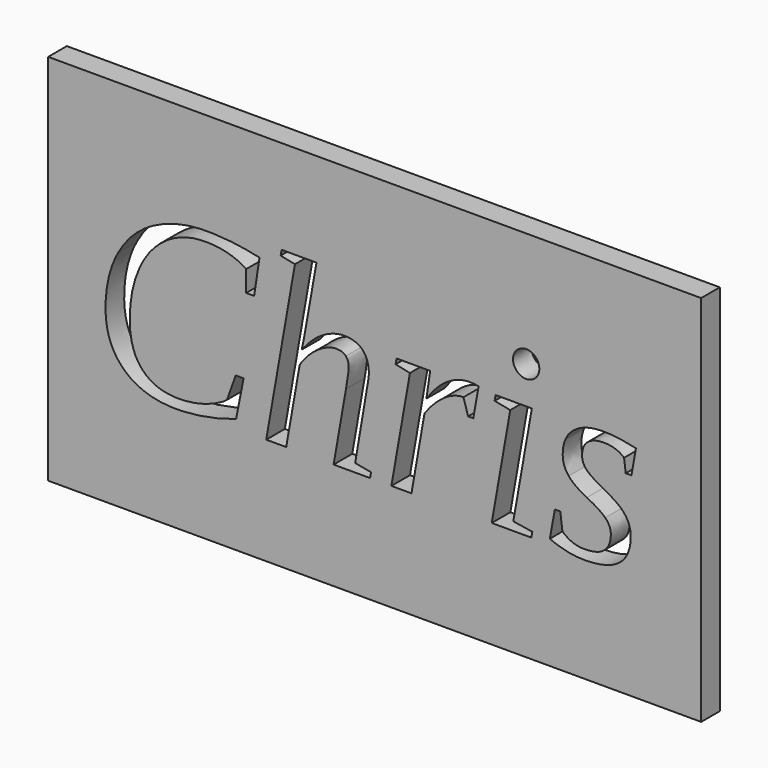
from build123d import *

# Parameters (mm, degrees)
F0_W     = 88.9
F0_H     = 50.8
F1_DEPTH = 3.175


with BuildPart() as f1:
    # F0 (on Front) → F1 (new body)
    with BuildSketch(Plane.XZ):
        with Locations((-44.45, 25.4)):
            Rectangle(F0_W, F0_H)
        with BuildLine():
            add(Edge.make_bspline(
                [(-34.643851095, 29.4662719552), (-33.1182674441, 30.4903661706), (-31.5979626294, 30.4903661706)],
                knots=[0, 0, 0, 1, 1, 1], degree=2))
            add(Edge.make_bspline(
                [(-31.5979626294, 30.4903661706), (-30.7744641881, 30.4903661706), (-30.2993689335, 30.3583952666)],
                knots=[0, 0, 0, 1, 1, 1], degree=2))
            Line((-30.2993689335, 30.3583952666), (-31.0225694878, 26.2989702579))
            Line((-31.0225694878, 26.2989702579), (-31.7299335335, 26.2989702579))
            Line((-31.7299335335, 26.2989702579), (-32.3581150368, 28.3946682143))
            add(Edge.make_bspline(
                [(-32.3581150368, 28.3946682143), (-33.6778240773, 28.3946682143), (-35.0899127507, 27.3890499254)],
                knots=[0, 0, 0, 1, 1, 1], degree=2))
            add(Edge.make_bspline(
                [(-35.0899127507, 27.3890499254), (-36.502001424, 26.3834316365), (-37.6686242158, 24.7311559178)],
                knots=[0, 0, 0, 1, 1, 1], degree=2))
            Line((-37.6686242158, 24.7311559178), (-39.4370343302, 14.5693963057))
            Line((-39.4370343302, 14.5693963057), (-42.1767502983, 14.5693963057))
            Line((-42.1767502983, 14.5693963057), (-39.6481877766, 28.9225518305))
            Line((-39.6481877766, 28.9225518305), (-41.5960783205, 29.3343010511))
            Line((-41.5960783205, 29.3343010511), (-41.4641074164, 30.07861695))
            Line((-41.4641074164, 30.07861695), (-36.8979141362, 30.07861695))
            Line((-36.8979141362, 30.07861695), (-37.4046824077, 26.5787485745))
            add(Edge.make_bspline(
                [(-37.4046824077, 26.5787485745), (-36.1694347458, 28.4421777397), (-34.643851095, 29.4662719552)],
                knots=[0, 0, 0, 1, 1, 1], degree=2))
        make_face(mode=Mode.SUBTRACT)
        Polygon((-23.051526883, 30.07861695), (-25.5748105685, 15.7254614252), (-22.988180849, 15.3137122046), (-23.1201517531, 14.5693963057), (-28.5151223108, 14.5693963057), (-25.9918386253, 28.9225518305), (-28.1192095986, 29.3343010511), (-27.9872386945, 30.07861695), align=None, mode=Mode.SUBTRACT)
        with BuildLine():
            add(Edge.make_bspline(
                [(-10.3823200939, 21.48203226), (-9.5904946696, 20.4605774626), (-9.5904946696, 19.1250319136)],
                knots=[0, 0, 0, 1, 1, 1], degree=2))
            add(Edge.make_bspline(
                [(-9.5904946696, 19.1250319136), (-9.5904946696, 16.6334212451), (-11.1741455182, 15.4351254363)],
                knots=[0, 0, 0, 1, 1, 1], degree=2))
            add(Edge.make_bspline(
                [(-11.1741455182, 15.4351254363), (-12.7577963669, 14.2368296275), (-15.9778864258, 14.2368296275)],
                knots=[0, 0, 0, 1, 1, 1], degree=2))
            add(Edge.make_bspline(
                [(-15.9778864258, 14.2368296275), (-18.2530648116, 14.2368296275), (-20.5968680676, 15.260923843)],
                knots=[0, 0, 0, 1, 1, 1], degree=2))
            Line((-20.5968680676, 15.260923843), (-19.9211770388, 18.9930610096))
            Line((-19.9211770388, 18.9930610096), (-19.17686114, 18.9930610096))
            Line((-19.17686114, 18.9930610096), (-18.8970828234, 16.728440296))
            add(Edge.make_bspline(
                [(-18.8970828234, 16.728440296), (-18.4694970943, 16.2691815499), (-17.6855899242, 15.9049418547)],
                knots=[0, 0, 0, 1, 1, 1], degree=2))
            add(Edge.make_bspline(
                [(-17.6855899242, 15.9049418547), (-16.9016827541, 15.5407021595), (-15.9092615556, 15.5407021595)],
                knots=[0, 0, 0, 1, 1, 1], degree=2))
            add(Edge.make_bspline(
                [(-15.9092615556, 15.5407021595), (-12.2985376208, 15.5407021595), (-12.2985376208, 18.4968504103)],
                knots=[0, 0, 0, 1, 1, 1], degree=2))
            add(Edge.make_bspline(
                [(-12.2985376208, 18.4968504103), (-12.2985376208, 19.4681562642), (-13.0666082824, 20.2283086715)],
                knots=[0, 0, 0, 1, 1, 1], degree=2))
            add(Edge.make_bspline(
                [(-13.0666082824, 20.2283086715), (-13.8346789439, 20.9884610788), (-15.5661372051, 21.8277960286)],
                knots=[0, 0, 0, 1, 1, 1], degree=2))
            add(Edge.make_bspline(
                [(-15.5661372051, 21.8277960286), (-17.2289705962, 22.6354579614), (-18.0392719471, 23.6173214876)],
                knots=[0, 0, 0, 1, 1, 1], degree=2))
            add(Edge.make_bspline(
                [(-18.0392719471, 23.6173214876), (-18.8495732979, 24.5991850137), (-18.8495732979, 25.9188940542)],
                knots=[0, 0, 0, 1, 1, 1], degree=2))
            add(Edge.make_bspline(
                [(-18.8495732979, 25.9188940542), (-18.8495732979, 28.0990533892), (-17.3794174268, 29.2947097799)],
                knots=[0, 0, 0, 1, 1, 1], degree=2))
            add(Edge.make_bspline(
                [(-17.3794174268, 29.2947097799), (-15.9092615556, 30.4903661706), (-13.3067953277, 30.4903661706)],
                knots=[0, 0, 0, 1, 1, 1], degree=2))
            add(Edge.make_bspline(
                [(-13.3067953277, 30.4903661706), (-11.4380873263, 30.4903661706), (-8.8831306239, 29.9096941928)],
                knots=[0, 0, 0, 1, 1, 1], degree=2))
            Line((-8.8831306239, 29.9096941928), (-9.4954756187, 26.4626141789))
            Line((-9.4954756187, 26.4626141789), (-10.2714645345, 26.4626141789))
            Line((-10.2714645345, 26.4626141789), (-10.4984544895, 28.2468608017))
            add(Edge.make_bspline(
                [(-10.4984544895, 28.2468608017), (-11.5383852134, 29.1706571301), (-13.2381704576, 29.1706571301)],
                knots=[0, 0, 0, 1, 1, 1], degree=2))
            add(Edge.make_bspline(
                [(-13.2381704576, 29.1706571301), (-14.5895525151, 29.1706571301), (-15.399853866, 28.5503938811)],
                knots=[0, 0, 0, 1, 1, 1], degree=2))
            add(Edge.make_bspline(
                [(-15.399853866, 28.5503938811), (-16.2101552169, 27.930130632), (-16.2101552169, 26.6262581)],
                knots=[0, 0, 0, 1, 1, 1], degree=2))
            add(Edge.make_bspline(
                [(-16.2101552169, 26.6262581), (-16.2101552169, 25.7394136247), (-15.5159882616, 25.0610831779)],
                knots=[0, 0, 0, 1, 1, 1], degree=2))
            add(Edge.make_bspline(
                [(-15.5159882616, 25.0610831779), (-14.8218213063, 24.3827527311), (-12.8897672709, 23.3956103688)],
                knots=[0, 0, 0, 1, 1, 1], degree=2))
            add(Edge.make_bspline(
                [(-12.8897672709, 23.3956103688), (-11.1741455182, 22.5034870574), (-10.3823200939, 21.48203226)],
                knots=[0, 0, 0, 1, 1, 1], degree=2))
        make_face(mode=Mode.SUBTRACT)
        with BuildLine():
            add(Edge.make_bspline(
                [(-67.3884718085, 14.6459394301), (-69.5739099796, 14.2579449722), (-71.442617981, 14.2579449722)],
                knots=[0, 0, 0, 1, 1, 1], degree=2))
            add(Edge.make_bspline(
                [(-71.442617981, 14.2579449722), (-75.9771382443, 14.2579449722), (-78.5347343648, 16.6334212451)],
                knots=[0, 0, 0, 1, 1, 1], degree=2))
            add(Edge.make_bspline(
                [(-78.5347343648, 16.6334212451), (-81.0923304853, 19.008897518), (-81.0923304853, 23.1950145946)],
                knots=[0, 0, 0, 1, 1, 1], degree=2))
            add(Edge.make_bspline(
                [(-81.0923304853, 23.1950145946), (-81.0923304853, 27.2861126202), (-79.3846269869, 30.4217413005)],
                knots=[0, 0, 0, 1, 1, 1], degree=2))
            add(Edge.make_bspline(
                [(-79.3846269869, 30.4217413005), (-77.6769234884, 33.5573699808), (-74.5333765539, 35.2492369708)],
                knots=[0, 0, 0, 1, 1, 1], degree=2))
            add(Edge.make_bspline(
                [(-74.5333765539, 35.2492369708), (-71.3898296194, 36.9411039607), (-67.3515199554, 36.9411039607)],
                knots=[0, 0, 0, 1, 1, 1], degree=2))
            add(Edge.make_bspline(
                [(-67.3515199554, 36.9411039607), (-63.8674880884, 36.9411039607), (-60.1247932494, 36.0964901748)],
                knots=[0, 0, 0, 1, 1, 1], degree=2))
            Line((-60.1247932494, 36.0964901748), (-60.8638303121, 31.2663550865))
            Line((-60.8638303121, 31.2663550865), (-61.9407128892, 31.2663550865))
            Line((-61.9407128892, 31.2663550865), (-61.9407128892, 34.1327631225))
            add(Edge.make_bspline(
                [(-61.9407128892, 34.1327631225), (-62.9595282685, 34.8454060044), (-64.4112082131, 35.2334004623)],
                knots=[0, 0, 0, 1, 1, 1], degree=2))
            add(Edge.make_bspline(
                [(-64.4112082131, 35.2334004623), (-65.8628881577, 35.6213949202), (-67.4465390063, 35.6213949202)],
                knots=[0, 0, 0, 1, 1, 1], degree=2))
            add(Edge.make_bspline(
                [(-67.4465390063, 35.6213949202), (-70.434360274, 35.6213949202), (-72.8019182927, 34.0271863992)],
                knots=[0, 0, 0, 1, 1, 1], degree=2))
            add(Edge.make_bspline(
                [(-72.8019182927, 34.0271863992), (-75.1694763114, 32.4329778783), (-76.4812670977, 29.5137814806)],
                knots=[0, 0, 0, 1, 1, 1], degree=2))
            add(Edge.make_bspline(
                [(-76.4812670977, 29.5137814806), (-77.793057884, 26.594585083), (-77.793057884, 22.8677267525)],
                knots=[0, 0, 0, 1, 1, 1], degree=2))
            add(Edge.make_bspline(
                [(-77.793057884, 22.8677267525), (-77.793057884, 19.3203488516), (-76.0695178771, 17.4648379406)],
                knots=[0, 0, 0, 1, 1, 1], degree=2))
            add(Edge.make_bspline(
                [(-76.0695178771, 17.4648379406), (-74.3459778702, 15.6093270297), (-71.1575608282, 15.6093270297)],
                knots=[0, 0, 0, 1, 1, 1], degree=2))
            add(Edge.make_bspline(
                [(-71.1575608282, 15.6093270297), (-69.2782951545, 15.6093270297), (-67.4808514413, 16.1688836628)],
                knots=[0, 0, 0, 1, 1, 1], degree=2))
            add(Edge.make_bspline(
                [(-67.4808514413, 16.1688836628), (-65.6834077281, 16.728440296), (-64.5590156256, 17.6047270989)],
                knots=[0, 0, 0, 1, 1, 1], degree=2))
            Line((-64.5590156256, 17.6047270989), (-63.3712774891, 20.9198362087))
            Line((-63.3712774891, 20.9198362087), (-62.2996737482, 20.9198362087))
            Line((-62.2996737482, 20.9198362087), (-63.3079314552, 15.7254614252))
            add(Edge.make_bspline(
                [(-63.3079314552, 15.7254614252), (-65.2030336374, 15.033933888), (-67.3884718085, 14.6459394301)],
                knots=[0, 0, 0, 1, 1, 1], degree=2))
        make_face(mode=Mode.SUBTRACT)
        with BuildLine():
            Line((-59.2168334296, 14.5693963057), (-55.3052158334, 36.8724790906))
            Line((-55.3052158334, 36.8724790906), (-57.2531063773, 37.2683918028))
            Line((-57.2531063773, 37.2683918028), (-57.1211354732, 38.0127077016))
            Line((-57.1211354732, 38.0127077016), (-52.3701829273, 38.0127077016))
            Line((-52.3701829273, 38.0127077016), (-54.117477697, 28.1782359316))
            Line((-54.117477697, 28.1782359316), (-54.3814195051, 26.9271517612))
            add(Edge.make_bspline(
                [(-54.3814195051, 26.9271517612), (-53.0617104645, 28.6586100224), (-51.5519633222, 29.5744880965)],
                knots=[0, 0, 0, 1, 1, 1], degree=2))
            add(Edge.make_bspline(
                [(-51.5519633222, 29.5744880965), (-50.0422161798, 30.4903661706), (-48.5905362352, 30.4903661706)],
                knots=[0, 0, 0, 1, 1, 1], degree=2))
            add(Edge.make_bspline(
                [(-48.5905362352, 30.4903661706), (-46.9277028442, 30.4903661706), (-46.0857284763, 29.590324605)],
                knots=[0, 0, 0, 1, 1, 1], degree=2))
            add(Edge.make_bspline(
                [(-46.0857284763, 29.590324605), (-45.2437541085, 28.6902830394), (-45.2437541085, 27.0063343036)],
                knots=[0, 0, 0, 1, 1, 1], degree=2))
            add(Edge.make_bspline(
                [(-45.2437541085, 27.0063343036), (-45.2437541085, 26.7793443487), (-45.3097395605, 26.2989702579)],
                knots=[0, 0, 0, 1, 1, 1], degree=2))
            add(Edge.make_bspline(
                [(-45.3097395605, 26.2989702579), (-45.3757250125, 25.8185961672), (-47.1071832737, 15.7096249167)],
                knots=[0, 0, 0, 1, 1, 1], degree=2))
            Line((-47.1071832737, 15.7096249167), (-44.9481392834, 15.3137122046))
            Line((-44.9481392834, 15.3137122046), (-45.0801101874, 14.5693963057))
            Line((-45.0801101874, 14.5693963057), (-50.0422161798, 14.5693963057))
            Line((-50.0422161798, 14.5693963057), (-48.3582674441, 24.1715992846))
            add(Edge.make_bspline(
                [(-48.3582674441, 24.1715992846), (-47.9834700766, 26.2672972409), (-47.9834700766, 26.9113152527)],
                knots=[0, 0, 0, 1, 1, 1], degree=2))
            add(Edge.make_bspline(
                [(-47.9834700766, 26.9113152527), (-47.9834700766, 27.6503523154), (-48.3793827888, 28.1122504796)],
                knots=[0, 0, 0, 1, 1, 1], degree=2))
            add(Edge.make_bspline(
                [(-48.3793827888, 28.1122504796), (-48.7752955009, 28.5741486438), (-49.6304669592, 28.5741486438)],
                knots=[0, 0, 0, 1, 1, 1], degree=2))
            add(Edge.make_bspline(
                [(-49.6304669592, 28.5741486438), (-50.8657146211, 28.5741486438), (-52.3015580572, 27.5447755922)],
                knots=[0, 0, 0, 1, 1, 1], degree=2))
            add(Edge.make_bspline(
                [(-52.3015580572, 27.5447755922), (-53.7374014933, 26.5154025406), (-54.6611978217, 25.0109342344)],
                knots=[0, 0, 0, 1, 1, 1], degree=2))
            Line((-54.6611978217, 25.0109342344), (-56.4929539699, 14.5693963057))
            Line((-56.4929539699, 14.5693963057), (-59.2168334296, 14.5693963057))
        make_face(mode=Mode.SUBTRACT)
        with BuildLine():
            add(Edge.make_bspline(
                [(-22.5605951199, 36.4132203445), (-22.0327115037, 35.8853367283), (-22.0327115037, 35.1410208294)],
                knots=[0, 0, 0, 1, 1, 1], degree=2))
            add(Edge.make_bspline(
                [(-22.0327115037, 35.1410208294), (-22.0327115037, 34.4125414391), (-22.5605951199, 33.8846578229)],
                knots=[0, 0, 0, 1, 1, 1], degree=2))
            add(Edge.make_bspline(
                [(-22.5605951199, 33.8846578229), (-23.0884787361, 33.3567742067), (-23.8275157988, 33.3567742067)],
                knots=[0, 0, 0, 1, 1, 1], degree=2))
            add(Edge.make_bspline(
                [(-23.8275157988, 33.3567742067), (-24.5559951892, 33.3567742067), (-25.0838788054, 33.8846578229)],
                knots=[0, 0, 0, 1, 1, 1], degree=2))
            add(Edge.make_bspline(
                [(-25.0838788054, 33.8846578229), (-25.6117624216, 34.4125414391), (-25.6117624216, 35.1410208294)],
                knots=[0, 0, 0, 1, 1, 1], degree=2))
            add(Edge.make_bspline(
                [(-25.6117624216, 35.1410208294), (-25.6117624216, 35.8853367283), (-25.0838788054, 36.4132203445)],
                knots=[0, 0, 0, 1, 1, 1], degree=2))
            add(Edge.make_bspline(
                [(-25.0838788054, 36.4132203445), (-24.5559951892, 36.9411039607), (-23.8275157988, 36.9411039607)],
                knots=[0, 0, 0, 1, 1, 1], degree=2))
            add(Edge.make_bspline(
                [(-23.8275157988, 36.9411039607), (-23.0884787361, 36.9411039607), (-22.5605951199, 36.4132203445)],
                knots=[0, 0, 0, 1, 1, 1], degree=2))
        make_face(mode=Mode.SUBTRACT)
    extrude(amount=F1_DEPTH)


solid = f1.part
